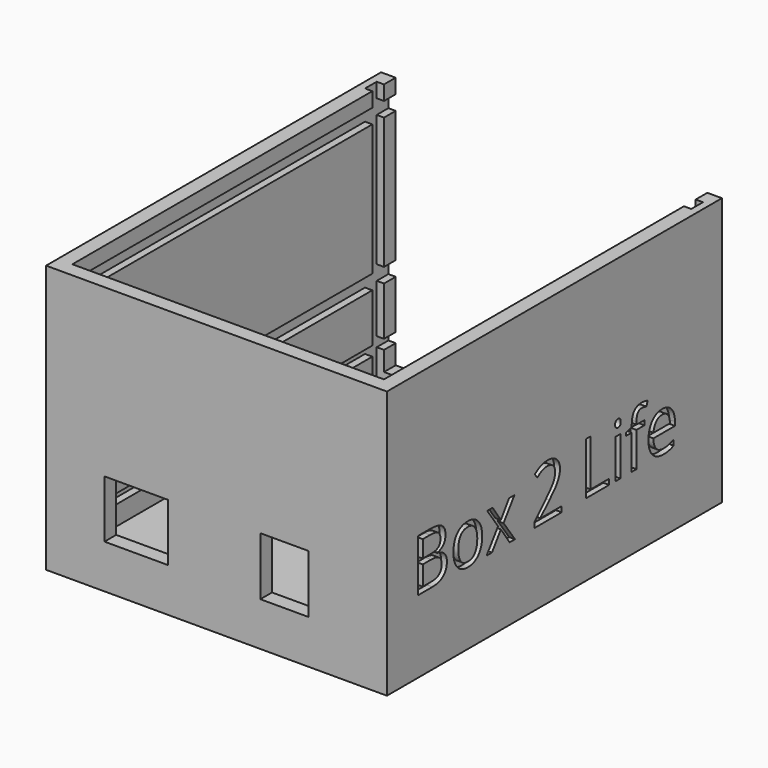
from build123d import *

# Parameters (mm, degrees)
F1_DEPTH      = 74
F2_W          = 70
F2_H          = 55
F2_W_2        = 13
F2_H_2        = 11.8
F2_W_3        = 9.93
F2_H_3        = 11.94
F3_DEPTH      = 3
F5_DEPTH      = 9
F7_W          = 3
F7_H          = 51.9999999739
F8_DEPTH      = 1.5
F10_W         = 3
F10_H         = 51.9999999739
F11_DEPTH     = 1.5
F12_W         = 66.9999999478
F12_H         = 3
F13_DEPTH     = 1.5
F14_TEXT_SIZE = 15.0348409079
F15_DEPTH     = 1.2


# Not quite as in the source:
# - Text() gives the source's letters only with a copy of the font that has no kerning and outlines rounded to 1/6400 em; it was checked with that copy


with BuildPart() as f1:
    # F0 (on Front) → F1 (new body)
    with BuildSketch(Plane.XZ):
        Polygon((0, 55), (0, 0), (70, 0), (70, 55), (66.9999999739, 55), (66.9999999739, 52), (68.4999999739, 52), (68.4999999739, 49), (66.9999999739, 49), (66.9999999739, 18.0000000261), (55.5400000261, 18.0000000261), (55.5400000261, 9.0000000261), (57.0400000261, 9.0000000261), (57.0400000261, 7.0000000261), (55.5400000261, 7.0000000261), (55.5400000261, 3.0000000261), (3.0000000261, 3.0000000261), (3.0000000261, 7.0000000261), (1.5000000261, 7.0000000261), (1.5000000261, 9.0000000261), (3.0000000261, 9.0000000261), (3.0000000261, 19.0000000261), (1.5000000261, 19.0000000261), (1.5000000261, 22.0000000261), (3.0000000261, 22.0000000261), (3.0000000261, 49), (1.5000000261, 49), (1.5000000261, 52), (3.0000000261, 52), (3.0000000261, 55), align=None)
    extrude(amount=-F1_DEPTH)

    # F2 (on face) → F3 (join)
    with BuildSketch(Plane.XZ):
        with Locations((35, 27.5)):
            Rectangle(F2_W, F2_H)
        with Locations((18.5000000261, 14.9000000261)):
            Rectangle(F2_W_2, F2_H_2, mode=Mode.SUBTRACT)
        with Locations((48.9650000261, 14.9700000261)):
            Rectangle(F2_W_3, F2_H_3, mode=Mode.SUBTRACT)
    extrude(amount=F3_DEPTH)

    # F4 (on face) → F5 (join)
    with BuildSketch(Plane(origin=(0, 74, 0), x_dir=(-1, 0, 0), z_dir=(0, 1, 0))):
        Polygon((-70, 55), (-70, 0), (0, 0), (0, 55), (-3.0000000261, 55), (-3.0000000261, 52), (-1.5000000261, 52), (-1.5000000261, 49), (-3.0000000261, 49), (-3.0000000261, 22.0000000261), (-1.5000000261, 22.0000000261), (-1.5000000261, 19.0000000261), (-3.0000000261, 19.0000000261), (-3.0000000261, 9.0000000261), (-1.5000000261, 9.0000000261), (-1.5000000261, 7.0000000261), (-3.0000000261, 7.0000000261), (-3.0000000261, 3.0000000261), (-55.5400000261, 3.0000000261), (-66.9999999739, 3.0000000261), (-66.9999999739, 18.0000000261), (-66.9999999739, 49), (-68.4999999739, 49), (-68.4999999739, 52), (-66.9999999739, 52), (-66.9999999739, 55), align=None)
    extrude(amount=F5_DEPTH)

    # F7 (on offset) → F8 (cut)
    with BuildSketch(Plane(origin=(66.9999999739, 0, 0), x_dir=(0, -1, 0), z_dir=(-1, 0, 0))):
        with Locations((-78.5, 29.000000013)):
            Rectangle(F7_W, F7_H)
    extrude(amount=-F8_DEPTH, mode=Mode.SUBTRACT)

    # F10 (on offset) → F11 (cut)
    with BuildSketch(Plane.YZ.offset(3.0000000261)):
        with Locations((78.5, 29.000000013)):
            Rectangle(F10_W, F10_H)
    extrude(amount=-F11_DEPTH, mode=Mode.SUBTRACT)

    # F12 (on face) → F13 (cut)
    with BuildSketch(Plane.XY.offset(3.0000000261)):
        with Locations((35, 78.5)):
            Rectangle(F12_W, F12_H)
    extrude(amount=-F13_DEPTH, mode=Mode.SUBTRACT)

    # F14 (on face) → F15 (cut)
    with BuildSketch(Plane.YZ.offset(70)):
        with Locations((3.4793014638, 14.9210998788)):
            Text('Box 2 Life', F14_TEXT_SIZE, font='Open Sans', text_align=(TextAlign.LEFT, TextAlign.BOTTOM))
    extrude(amount=-F15_DEPTH, mode=Mode.SUBTRACT)


solid = f1.part
